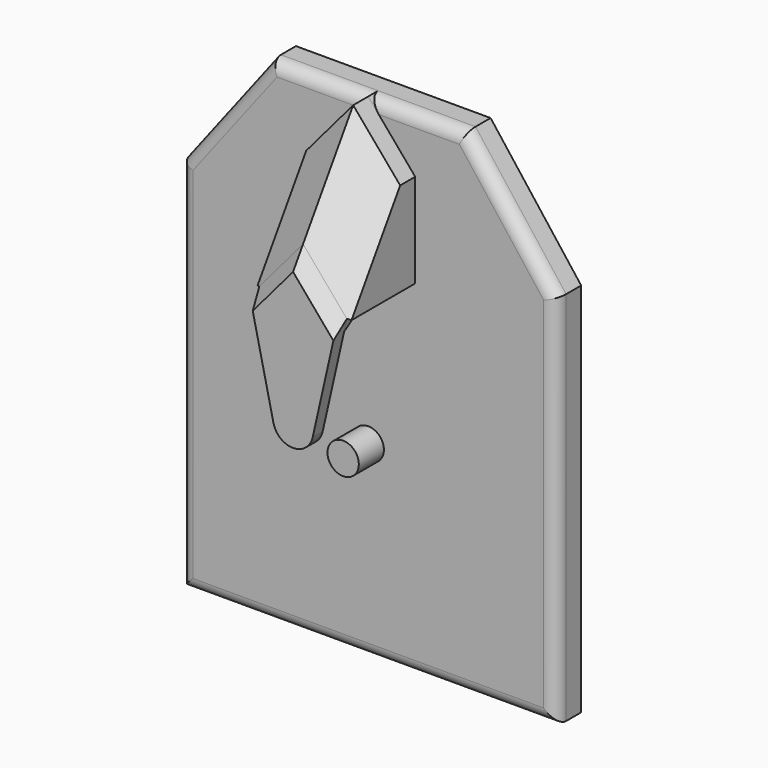
from build123d import *

# Parameters (mm, degrees)
F0_W          = 78.9395868778
F0_H          = 47.8476444364
F1_DEPTH      = 12.7
F2_R          = 6.35
F3_DEPTH      = 12.7
F5_DEPTH      = 33.02
F6_SIZE       = 25.4
F8_DEPTH      = 5.08
F9_T4_ANGLE   = 53.6437900891
F9_T7_DEPTH   = 53.5623511666
F9_T9_DEPTH   = 53.5623511666
F10_T1_DEPTH  = 85.7200228127
F10_T3_DEPTH  = 177.8
F10_T5_DEPTH  = 85.7200228127
F10_T7_DEPTH  = 177.8
F10_T12_DEPTH = 52.1697934389
F10_T17_DEPTH = 52.1697934389


# Not quite as in the source:
# - a fillet or chamfer that OpenCascade refuses, or shapes differently, is made with other operations: its cross-section is extruded or revolved along the edge and cut away or added


with BuildPart() as f1:
    # F0 (on Front) → F1 (new body)
    with BuildSketch(Plane.XZ):
        Polygon((-39.4697934389, 124.0476444364), (-76.2, 76.2), (-39.4697934389, 76.2), align=None)
        Polygon((-39.4697934389, 76.2), (-76.2, 76.2), (-76.2, -76.2), (76.2, -76.2), (76.2, 76.2), (39.4697934389, 76.2), (39.4697934389, 28.3523555636), (-39.4697934389, 28.3523555636), align=None)
        with Locations((0, 100.1238222182)):
            Rectangle(F0_W, F0_H)
        Polygon((39.4697934389, 124.0476444364), (39.4697934389, 76.2), (76.2, 76.2), align=None)
        with Locations((0, 52.2761777818)):
            Rectangle(F0_W, F0_H)
    extrude(amount=F1_DEPTH)

    # F2 (on face) → F3 (join)
    with BuildSketch(Plane.XZ.offset(12.7)):
        Circle(F2_R)
    extrude(amount=F3_DEPTH)

    # F4 (on face) → F5 (join)
    with BuildSketch(Plane.XZ.offset(12.7)):
        Polygon((0, 124.0476444364), (-19.05, 101.6), (19.05, 101.6), align=None)
        with BuildLine():
            Line((19.05, 101.6), (-19.05, 101.6))
            Line((-19.05, 101.6), (-19.05, 63.5))
            ThreePointArc((-19.05, 63.5), (0, 66.2959463316), (19.05, 63.5))
            Line((19.05, 63.5), (19.05, 101.6))
        make_face()
    extrude(amount=F5_DEPTH)

    # F6
    f6_edges = [f1.edges().sort_by_distance(p)[0] for p in [
        (9.525, -45.72, 112.823822),
        (-9.525, -45.72, 112.823822),
    ]]
    chamfer(f6_edges, length=F6_SIZE)

    # F7 (on face) → F8 (join)
    with BuildSketch(Plane.XZ.offset(45.72)):
        with BuildLine():
            ThreePointArc((7.9480178428, 20.4315265516), (8.0977413026, 21.3227137731), (8.1478546035, 22.225))
            ThreePointArc((8.1478546035, 22.225), (-0.9022862269, 30.3227413026), (-7.9480178428, 20.4315265516))
            ThreePointArc((-7.9480178428, 20.4315265516), (0, 14.0771453965), (7.9480178428, 20.4315265516))
        make_face()
        with BuildLine():
            ThreePointArc((-7.9480178428, 20.4315265516), (-0.9022862269, 30.3227413026), (8.1478546035, 22.225))
            ThreePointArc((8.1478546035, 22.225), (8.0977413026, 21.3227137731), (7.9480178428, 20.4315265516))
            Line((7.9480178428, 20.4315265516), (17.7511165922, 63.8752718956))
            ThreePointArc((17.7511165922, 63.8752718956), (0, 66.2959463316), (-17.7511165922, 63.8752718956))
            Line((-17.7511165922, 63.8752718956), (-7.9480178428, 20.4315265516))
        make_face()
        with BuildLine():
            Line((0, 84.7923718226), (-17.7511165922, 63.8752718956))
            ThreePointArc((-17.7511165922, 63.8752718956), (0, 66.2959463316), (17.7511165922, 63.8752718956))
            Line((17.7511165922, 63.8752718956), (0, 84.7923718226))
        make_face()
    extrude(amount=F8_DEPTH)

    # F9: chamfer of 5.08 on 3 edges, made by hand


with BuildPart() as f9_tool2:
    # F9_s3 → F9_t4 (revolve)
    with BuildSketch(Plane(origin=(0, 0, 0), x_dir=(0, 1, 0), z_dir=(-0.8924134547, 0, -0.4512186011))):
        Polygon((-40.64, -66.2959463316), (-45.72, -61.2159463316), (-45.72, -66.2959463316), align=None)
    revolve(axis=Axis((0, -45.72, 0), (0, 1, 0)), revolution_arc=F9_T4_ANGLE)

    split(bisect_by=Plane(origin=(-3.1759235814, 0, -0.7166484437), x_dir=(0, 1, 0), z_dir=(0.9754736958, 0, 0.2201160349)), keep=Keep.TOP)

    split(bisect_by=Plane(origin=(3.1759235814, 0, -0.7166484437), x_dir=(0, 1, 0), z_dir=(-0.9754736958, 0, 0.2201160349)), keep=Keep.TOP)


with BuildPart() as f1_1:
    add(f1.part)

    # F9_t1: union F9_tool2
    add(f9_tool2.part)

    # F9_s8 → F9_t7 (cut)
    with BuildSketch(Plane(origin=(50.284672357, 0, 59.2531467543), x_dir=(0, 1, 0), z_dir=(-0.6470468375, 0, -0.7624502542))):
        Polygon((-45.72, -54.864636032), (-50.8, -49.784636032), (-50.8, -54.864636032), align=None)
    extrude(amount=F9_T7_DEPTH, mode=Mode.SUBTRACT)

    # F9_s10 → F9_t9 (cut)
    with BuildSketch(Plane(origin=(-15.6273224256, 0, 18.4145184935), x_dir=(0, 1, 0), z_dir=(-0.6470468375, 0, 0.7624502542))):
        Polygon((-45.72, -54.864636032), (-50.8, -49.784636032), (-50.8, -54.864636032), align=None)
    extrude(amount=F9_T9_DEPTH, mode=Mode.SUBTRACT)

    # F10: fillet of radius 5.08 on 7 edges, made by hand

    # F10_s2 → F10_t1 (cut)
    with BuildSketch(Plane(origin=(-0.8185365807, 0, 1.0662898725), x_dir=(0, 1, 0), z_dir=(-0.6089222923, 0, 0.7932298797))):
        with BuildLine():
            ThreePointArc((-12.7, -101.7639955007), (-11.2121024484, -105.3560979491), (-7.62, -106.8439955007))
            Line((-7.62, -106.8439955007), (-12.7, -106.8439955007))
            Line((-12.7, -106.8439955007), (-12.7, -101.7639955007))
        make_face()
    extrude(amount=F10_T1_DEPTH, mode=Mode.SUBTRACT)

    # F10_s4 → F10_t3 (cut)
    with BuildSketch(Plane.XY.offset(-88.9)):
        with BuildLine():
            ThreePointArc((71.12, -12.7), (74.7121024484, -11.2121024484), (76.2, -7.62))
            Line((76.2, -7.62), (76.2, -12.7))
            Line((76.2, -12.7), (71.12, -12.7))
        make_face()
        with BuildLine():
            ThreePointArc((-71.12, -12.7), (-74.7121024484, -11.2121024484), (-76.2, -7.62))
            Line((-76.2, -7.62), (-76.2, -12.7))
            Line((-76.2, -12.7), (-71.12, -12.7))
        make_face()
    extrude(amount=F10_T3_DEPTH, mode=Mode.SUBTRACT)

    # F10_s6 → F10_t5 (cut)
    with BuildSketch(Plane(origin=(53.0153693655, 0, 69.0619732521), x_dir=(0, 1, 0), z_dir=(-0.6089222923, 0, -0.7932298797))):
        with BuildLine():
            ThreePointArc((-12.7, -101.7639955007), (-11.2121024484, -105.3560979491), (-7.62, -106.8439955007))
            Line((-7.62, -106.8439955007), (-12.7, -106.8439955007))
            Line((-12.7, -106.8439955007), (-12.7, -101.7639955007))
        make_face()
    extrude(amount=F10_T5_DEPTH, mode=Mode.SUBTRACT)

    # F10_s8 → F10_t7 (cut)
    with BuildSketch(Plane.YZ.offset(-88.9)):
        with BuildLine():
            ThreePointArc((-12.7, -71.12), (-11.2121024484, -74.7121024484), (-7.62, -76.2))
            Line((-7.62, -76.2), (-12.7, -76.2))
            Line((-12.7, -76.2), (-12.7, -71.12))
        make_face()
    extrude(amount=F10_T7_DEPTH, mode=Mode.SUBTRACT)


with BuildPart() as f10_tool10:
    # F10_s11 → F10_t12 (new body)
    with BuildSketch(Plane.YZ.offset(52.1697934389)):
        with BuildLine():
            ThreePointArc((-12.7, 118.9676444364), (-11.2121024484, 122.5597468848), (-7.62, 124.0476444364))
            Line((-7.62, 124.0476444364), (-12.7, 124.0476444364))
            Line((-12.7, 124.0476444364), (-12.7, 118.9676444364))
        make_face()
    extrude(amount=-F10_T12_DEPTH)

    split(bisect_by=Plane(origin=(61.1977921432, 0, 51.9349789077), x_dir=(0, 1, 0), z_dir=(0.7624502542, 0, 0.6470468375)), keep=Keep.TOP)


with BuildPart() as f1_2:
    add(f1_1.part)

    # F10_t9: cut F10_tool10
    add(f10_tool10.part, mode=Mode.SUBTRACT)


with BuildPart() as f10_tool15:
    # F10_s16 → F10_t17 (new body)
    with BuildSketch(Plane.YZ):
        with BuildLine():
            ThreePointArc((-12.7, 118.9676444364), (-11.2121024484, 122.5597468848), (-7.62, 124.0476444364))
            Line((-7.62, 124.0476444364), (-12.7, 124.0476444364))
            Line((-12.7, 124.0476444364), (-12.7, 118.9676444364))
        make_face()
    extrude(amount=-F10_T17_DEPTH)

    split(bisect_by=Plane(origin=(-61.1977921432, 0, 51.9349789077), x_dir=(0, 1, 0), z_dir=(-0.7624502542, 0, 0.6470468375)), keep=Keep.TOP)


with BuildPart() as f1_3:
    add(f1_2.part)

    # F10_t14: cut F10_tool15
    add(f10_tool15.part, mode=Mode.SUBTRACT)


solid = f1_3.part
